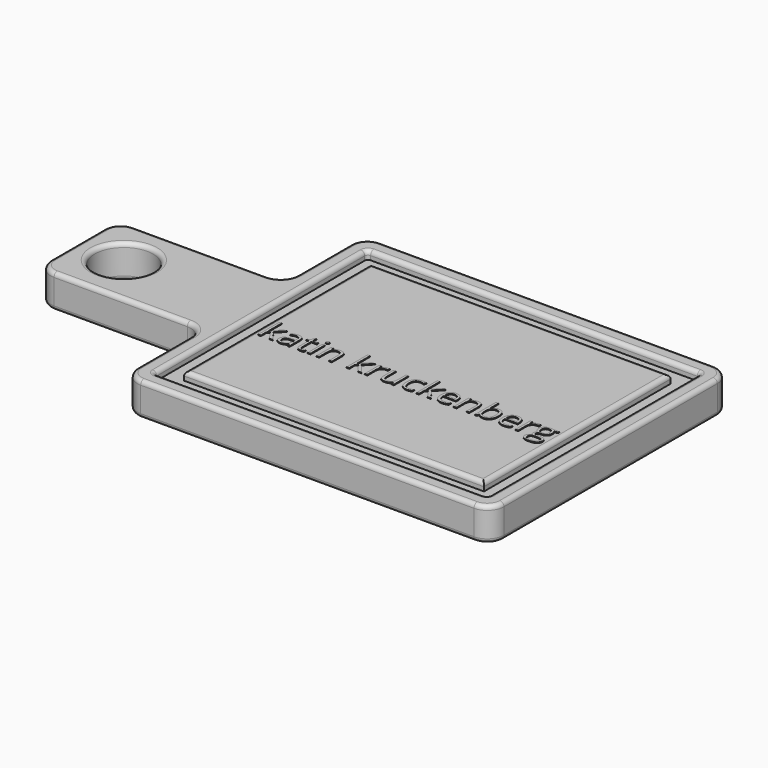
from build123d import *

# Parameters (mm, degrees)
F0_W         = 127
F0_H         = 76.2
F1_DEPTH     = 25.4
F2_R         = 22.225
F3_DEPTH     = 25.4
F4_W         = 254.0000078201
F4_H         = 203.2000078201
F4_W_2       = 228.5999950886
F4_H_2       = 177.7999950886
F5_DEPTH     = 6.35
F6_R         = 2.54
F7_R         = 12.7
F8_R         = 3.175
F9_TEXT_SIZE = 26.2891355592
F10_DEPTH    = 0.508


# Not quite as in the source:
# - Text() gives the source's letters only with a copy of the font that has no kerning and outlines rounded to 1/6400 em; it was checked with that copy


with BuildPart() as f1:
    # F0 (on Top) → F1 (new body)
    with BuildSketch(Plane.XY):
        Polygon((0, 76.2), (0, 0), (279.4, 0), (279.4, 228.6), (0, 228.6), (0, 152.4), align=None)
        with Locations((-63.5, 114.3)):
            Rectangle(F0_W, F0_H)
    extrude(amount=F1_DEPTH)

    # F2 (on face) → F3 (cut)
    with BuildSketch(Plane.XY.offset(25.4)):
        with Locations((-92.0807732044, 114.935)):
            Circle(F2_R)
    extrude(amount=-F3_DEPTH, mode=Mode.SUBTRACT)

    # F4 (on face) → F5 (cut)
    with BuildSketch(Plane.XY.offset(25.4)):
        with Locations((139.7, 114.3)):
            Rectangle(F4_W, F4_H)
        with Locations((139.7, 114.3)):
            Rectangle(F4_W_2, F4_H_2, mode=Mode.SUBTRACT)
    extrude(amount=-F5_DEPTH, mode=Mode.SUBTRACT)

    # F6
    f6_edges = [f1.edges().sort_by_distance(p)[0] for p in [
        (266.700004, 215.900004, 22.225),
        (12.699996, 215.900004, 22.225),
        (12.699996, 12.699996, 22.225),
        (266.700004, 12.699996, 22.225),
    ]]
    fillet(f6_edges, radius=F6_R)

    # F7
    f7_edges = [f1.edges().sort_by_distance(p)[0] for p in [
        (0, 0, 12.7),
        (-127, 76.2, 12.7),
        (279.4, 0, 12.7),
        (279.4, 228.6, 12.7),
        (0, 228.6, 12.7),
        (-127, 152.4, 12.7),
        (0, 152.4, 12.7),
        (0, 76.2, 12.7),
    ]]
    fillet(f7_edges, radius=F7_R)

    # F8
    f8_edges = [f1.edges().sort_by_distance(p)[0] for p in [
        (0, 38.1, 25.4),
        (-3.719744, 72.480256, 25.4),
        (3.719744, 3.719744, 25.4),
        (-63.5, 76.2, 25.4),
        (139.7, 0, 25.4),
        (-123.280256, 79.919744, 25.4),
        (275.680256, 3.719744, 25.4),
        (-127, 114.3, 25.4),
        (279.4, 114.3, 25.4),
        (-123.280256, 148.680256, 25.4),
        (275.680256, 224.880256, 25.4),
        (-63.5, 152.4, 25.4),
        (139.7, 228.6, 25.4),
        (-3.719744, 156.119744, 25.4),
        (3.719744, 224.880256, 25.4),
        (0, 190.5, 25.4),
        (139.7, 215.900004, 25.4),
        (265.956055, 215.156055, 25.4),
        (13.443945, 215.156055, 25.4),
        (266.700004, 114.3, 25.4),
        (12.699996, 114.3, 25.4),
        (265.956055, 13.443945, 25.4),
        (13.443945, 13.443945, 25.4),
        (139.7, 12.699996, 25.4),
        (-114.305773, 114.935, 25.4),
        (25.400002, 114.3, 25.4),
        (139.7, 203.199998, 25.4),
        (253.999998, 114.3, 25.4),
        (139.7, 25.400002, 25.4),
        (0, 38.1, 0),
        (-3.719744, 72.480256, 0),
        (3.719744, 3.719744, 0),
        (-63.5, 76.2, 0),
        (139.7, 0, 0),
        (-123.280256, 79.919744, 0),
        (275.680256, 3.719744, 0),
        (-127, 114.3, 0),
        (279.4, 114.3, 0),
        (-123.280256, 148.680256, 0),
        (275.680256, 224.880256, 0),
        (-63.5, 152.4, 0),
        (139.7, 228.6, 0),
        (-3.719744, 156.119744, 0),
        (3.719744, 224.880256, 0),
        (0, 190.5, 0),
        (-114.305773, 114.935, 0),
    ]]
    fillet(f8_edges, radius=F8_R)

    # F9 (on face) → F10 (join)
    with BuildSketch(Plane.XY.offset(25.4)):
        with Locations((28.5750024557, 89.2313917652)):
            Text('katin kruckenberg', F9_TEXT_SIZE, font='Open Sans', text_align=(TextAlign.LEFT, TextAlign.BOTTOM))
    extrude(amount=F10_DEPTH)


solid = f1.part
